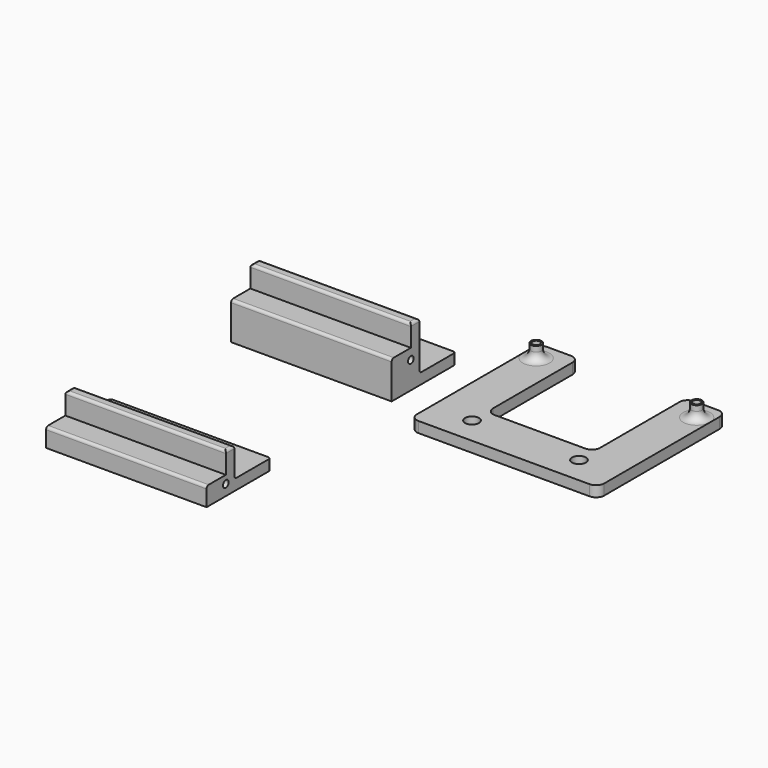
from build123d import *

# Parameters (mm, degrees)
F0_W      = 60
F0_H      = 17
F0_R      = 2.6
F0_H_2    = 13
F1_DEPTH  = 4
F2_DEPTH  = 10
F3_W      = 60
F3_H      = 4
F4_DEPTH  = 8
F5_R      = 1.3
F6_DEPTH  = 60.001
F7_R      = 1
F8_W      = 60
F8_H      = 13
F8_H_2    = 17
F8_R      = 2.6
F9_DEPTH  = 4
F10_DEPTH = 3
F11_W     = 60
F11_H     = 4
F12_DEPTH = 8
F13_R     = 1.3
F14_DEPTH = 60.40970592
F15_R     = 1
F16_R     = 2.6
F16_R_2   = 2
F16_R_3   = 1.4
F17_DEPTH = 4
F18_DEPTH = 5
F19_R     = 2.99999


# Not quite as in the source:
# - a fillet or chamfer is up to 0.001 mm smaller than in the source, because OpenCascade refuses the exact size


with BuildPart() as f1:
    # F0 (on Top) → F1 (new body)
    with BuildSketch(Plane.XY):
        with Locations((-40.7936765254, 52.8680981398)):
            Rectangle(F0_W, F0_H)
        with Locations((-55.7936765254, 51.3680981398)):
            Circle(F0_R, mode=Mode.SUBTRACT)
        with Locations((-25.7936765254, 51.3680981398)):
            Circle(F0_R, mode=Mode.SUBTRACT)
        with Locations((-40.7936765254, 37.8680981398)):
            Rectangle(F0_W, F0_H_2)
    extrude(amount=-F1_DEPTH)

    # F0 (on Top) → F2 (join)
    with BuildSketch(Plane.XY):
        with Locations((-40.7936765254, 37.8680981398)):
            Rectangle(F0_W, F0_H_2)
    extrude(amount=F2_DEPTH)

    # F3 (on face) → F4 (join)
    with BuildSketch(Plane.XY.offset(10)):
        with Locations((-40.7936765254, 42.3680981398)):
            Rectangle(F3_W, F3_H)
    extrude(amount=F4_DEPTH)

    # F5 (on face) → F6 (cut, through all)
    with BuildSketch(Plane.YZ.offset(-10.7936765254)):
        with Locations((40.3680981398, 6)):
            Circle(F5_R)
    extrude(amount=-F6_DEPTH, mode=Mode.SUBTRACT)

    # F7
    f7_edges = [f1.edges().sort_by_distance(p)[0] for p in [
        (-40.793677, 44.368098, 0),
        (-70.793677, 61.368098, -2),
        (-10.793677, 61.368098, -2),
        (-10.793677, 42.368098, 18),
        (-70.793677, 42.368098, 18),
        (-40.793677, 40.368098, 18),
        (-40.793677, 44.368098, 18),
        (-40.793677, 31.368098, 10),
    ]]
    fillet(f7_edges, radius=F7_R)


with BuildPart() as f9:
    # F8 (on Top) → F9 (new body)
    with BuildSketch(Plane.XY):
        with Locations((-41.2023824453, -48.0929382443)):
            Rectangle(F8_W, F8_H)
        with Locations((-41.2023824453, -33.0929382443)):
            Rectangle(F8_W, F8_H_2)
        with Locations((-56.2023824453, -34.5929382443)):
            Circle(F8_R, mode=Mode.SUBTRACT)
        with Locations((-26.2023824453, -34.5929382443)):
            Circle(F8_R, mode=Mode.SUBTRACT)
    extrude(amount=-F9_DEPTH)

    # F8 (on Top) → F10 (join)
    with BuildSketch(Plane.XY):
        with Locations((-41.2023824453, -48.0929382443)):
            Rectangle(F8_W, F8_H)
    extrude(amount=F10_DEPTH)

    # F11 (on face) → F12 (join)
    with BuildSketch(Plane.XY.offset(3)):
        with Locations((-41.2023824453, -43.5929382443)):
            Rectangle(F11_W, F11_H)
    extrude(amount=F12_DEPTH)

    # F13 (on face) → F14 (cut, through all)
    with BuildSketch(Plane(origin=(-71.2023824453, 0, 0), x_dir=(0, -1, 0), z_dir=(-1, 0, 0))):
        with Locations((45.5929382443, 0)):
            Circle(F13_R)
    extrude(amount=-F14_DEPTH, mode=Mode.SUBTRACT)

    # F15
    f15_edges = [f9.edges().sort_by_distance(p)[0] for p in [
        (-41.202382, -41.592938, 0),
        (-71.202382, -24.592938, -2),
        (-11.202382, -24.592938, -2),
        (-11.202382, -43.592938, 11),
        (-71.202382, -43.592938, 11),
        (-41.202382, -45.592938, 11),
        (-41.202382, -41.592938, 11),
        (-41.202382, -54.592938, 3),
    ]]
    fillet(f15_edges, radius=F15_R)


with BuildPart() as f17:
    # F16 (on Top) → F17 (new body)
    with BuildSketch(Plane.XY):
        Polygon((19.8487690091, 80.6387767196), (4.8487690091, 80.6387767196), (4.8487690091, 20.6387767196), (74.8487690091, 20.6387767196), (74.8487690091, 80.6387767196), (59.8487690091, 80.6387767196), (59.8487690091, 37.4572774023), (19.8487690091, 37.4572774023), align=None)
        with Locations((19.8487690091, 30.6387767196)):
            Circle(F16_R, mode=Mode.SUBTRACT)
        with Locations((59.8487690091, 30.6387767196)):
            Circle(F16_R, mode=Mode.SUBTRACT)
        with Locations((9.8487690091, 73.1387767196)):
            Circle(F16_R_2, mode=Mode.SUBTRACT)
        with Locations((69.8487690091, 73.1387767196)):
            Circle(F16_R_2, mode=Mode.SUBTRACT)
        with Locations((9.8487690091, 73.1387767196)):
            Circle(F16_R_2)
        with Locations((9.8487690091, 73.1387767196)):
            Circle(F16_R_3, mode=Mode.SUBTRACT)
        with Locations((69.8487690091, 73.1387767196)):
            Circle(F16_R_2)
        with Locations((69.8487690091, 73.1387767196)):
            Circle(F16_R_3, mode=Mode.SUBTRACT)
    extrude(amount=-F17_DEPTH)

    # F16 (on Top) → F18 (join)
    with BuildSketch(Plane.XY):
        with Locations((69.8487690091, 73.1387767196)):
            Circle(F16_R_2)
        with Locations((69.8487690091, 73.1387767196)):
            Circle(F16_R_3, mode=Mode.SUBTRACT)
        with Locations((9.8487690091, 73.1387767196)):
            Circle(F16_R_2)
        with Locations((9.8487690091, 73.1387767196)):
            Circle(F16_R_3, mode=Mode.SUBTRACT)
    extrude(amount=F18_DEPTH)

    # F19 (radius 3 in the source; OpenCascade refuses exactly that, so slightly less here)
    f19_edges = [f17.edges().sort_by_distance(p)[0] for p in [
        (4.848769, 80.638777, -2),
        (19.848769, 80.638777, -2),
        (59.848769, 80.638777, -2),
        (74.848769, 80.638777, -2),
        (19.848769, 37.457277, -2),
        (59.848769, 37.457277, -2),
        (4.848769, 20.638777, -2),
        (74.848769, 20.638777, -2),
        (7.848769, 73.138777, 0),
        (67.848769, 73.138777, 0),
    ]]
    fillet(f19_edges, radius=F19_R)


solid = Compound([f1.part, f9.part, f17.part])
